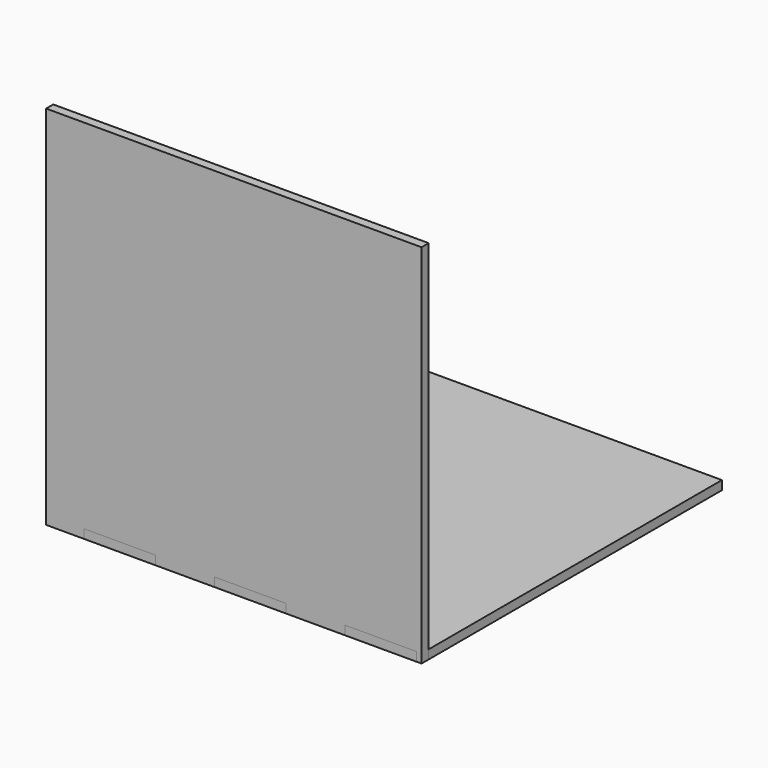
from build123d import *

# Parameters (mm, degrees)
F0_W          = 133.35
F0_H          = 133.35
F1_DEPTH      = 3.175
F2_W          = 133.35
F2_H          = 3.175
F3_DEPTH      = 127
F3_DEPTH_BACK = 3.175
F4_W          = 25.4
F4_H          = 3.175
F5_DEPTH      = 25.4


# Not quite as in the source:
# - a length typed as a fraction of an inch, garbled in the dataset ("3 / 203.2 mm" for 3/8 in), is restored


with BuildPart() as f1:
    # F0 (on Top) → F1 (new body)
    with BuildSketch(Plane.XY):
        with Locations((3.992497921, 1.1885885367)):
            Rectangle(F0_W, F0_H)
    extrude(amount=-F1_DEPTH)


with BuildPart() as f3:
    # F2 (on Top) → F3 (new body, two sides)
    with BuildSketch(Plane.XY) as f3_sk:
        with Locations((3.992497921, -63.8989114633)):
            Rectangle(F2_W, F2_H)
    extrude(amount=F3_DEPTH)
    extrude(f3_sk.sketch, amount=-F3_DEPTH_BACK)

    # F4 (on face) → F5 (cut)
    with BuildSketch(Plane.XZ.offset(65.4864114633)):
        with Locations((-36.5941066623, -1.5875)):
            Rectangle(F4_W, F4_H)
        with Locations((9.7608933377, -1.5875)):
            Rectangle(F4_W, F4_H)
        with Locations((56.1158933377, -1.5875)):
            Rectangle(F4_W, F4_H)
    extrude(amount=-F5_DEPTH, mode=Mode.SUBTRACT)


solid = Compound([f1.part, f3.part])
